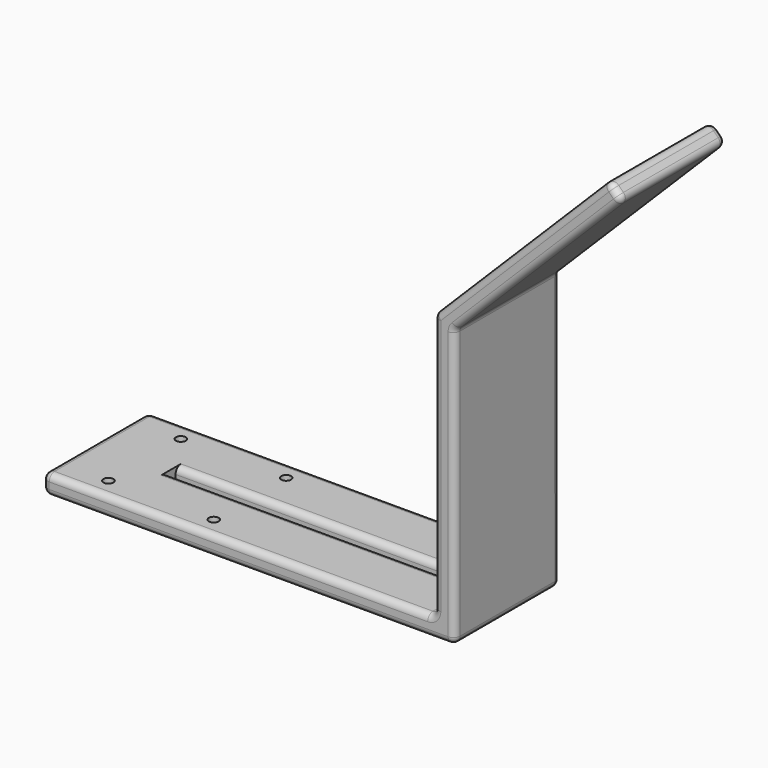
from build123d import *

# Parameters (mm, degrees)
F1_DEPTH       = 40
F3_D           = 3
F3_DEPTH       = 40
F3_CSINK_D     = 6
F3_CSINK_ANGLE = 90
F3_TIP         = 0.9012909285
F4_START       = -2.5
F2_W           = 98.723
F2_H           = 3.5
F4_DEPTH       = 98.5
F5_R           = 2


with BuildPart() as f1:
    # F0 (on Front) → F1 (new body)
    with BuildSketch(Plane.XZ):
        Polygon((53.7955448006, 85.2875881677), (53.7992331499, 4.6113628414), (-65.2007668501, 4.6113628414), (-65.2007668501, -1.3886371586), (60.0222331499, -1.3886371586), (60.0183739277, 83.0251359205), (111.0902979443, 134.055520892), (106.8493191704, 138.2998228416), align=None)
    extrude(amount=F1_DEPTH)

    # F3
    with Locations(Plane(origin=(0, 0, -1.3886371586), x_dir=(1, 0, 0), z_dir=(0, 0, -1))):
        with Locations((-50.2007668501, 33.75), (-50.2007668501, 6.25), (-18.2007668501, 6.25), (-18.2007668501, 33.75)):
            CounterSinkHole(F3_D / 2, F3_CSINK_D / 2, depth=F3_DEPTH, counter_sink_angle=F3_CSINK_ANGLE)
            with Locations((0, 0, -(F3_DEPTH + F3_TIP / 2))):  # 118° drill point
                Cone(0, F3_D / 2, F3_TIP, mode=Mode.SUBTRACT)

    # F2 (on face) → F4 (cut)
    with BuildSketch(Plane(origin=(0, 0, -1.3886371586), x_dir=(1, 0, 0), z_dir=(0, 0, -1)).offset(F4_START)):
        with Locations((7.1607331499, 20)):
            Rectangle(F2_W, F2_H)
    extrude(amount=-F4_DEPTH, mode=Mode.SUBTRACT)

    # F5
    f5_edges = [f1.edges().sort_by_distance(p)[0] for p in [
        (53.797389, -21.75, 44.949476),
        (53.799233, -30.875, 4.611363),
        (53.797389, -40, 44.949476),
        (53.795545, -30.875, 85.287588),
        (53.797389, 0, 44.949476),
        (53.799233, -9.125, 4.611363),
        (53.797389, -18.25, 44.949476),
        (53.795545, -9.125, 85.287588),
        (-65.200767, -20, 4.611363),
        (-65.200767, -20, -1.388637),
        (-65.200767, 0, 1.611363),
        (-65.200767, -40, 1.611363),
        (-5.700767, 0, 4.611363),
        (-2.589267, 0, -1.388637),
        (60.020304, 0, 40.818249),
        (85.554336, 0, 108.540328),
        (108.969809, 0, 136.177672),
        (80.322432, 0, 111.793706),
        (-5.700767, -40, 4.611363),
        (-2.589267, -40, -1.388637),
        (60.020304, -40, 40.818249),
        (85.554336, -40, 108.540328),
        (108.969809, -40, 136.177672),
        (80.322432, -40, 111.793706),
        (55.158889, -18.25, 86.649865),
        (56.522233, -20, 88.012142),
        (55.158889, -21.75, 86.649865),
        (106.849319, -20, 138.299823),
        (111.090298, -20, 134.055521),
        (60.022233, -20, -1.388637),
        (60.018374, -20, 83.025136),
        (5.799233, -21.75, 4.611363),
        (5.799233, -18.25, 4.611363),
    ]]
    fillet(f5_edges, radius=F5_R)


solid = f1.part
